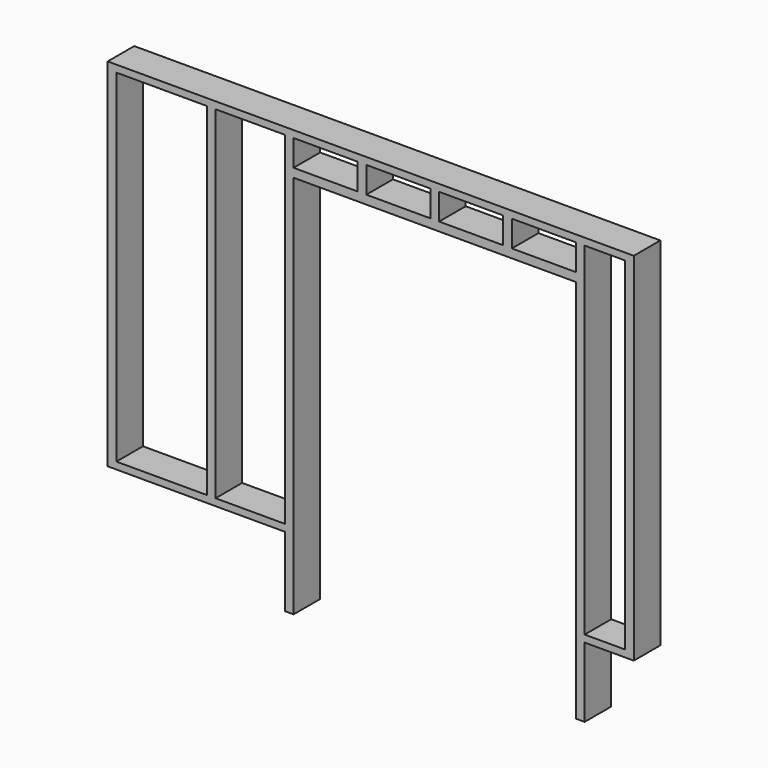
from build123d import *

# Parameters (mm, degrees)
F0_W     = 1014
F0_H     = 40
F1_DEPTH = 190
F0_W_2   = 3011
F2_DEPTH = 190
F3_W     = 50
F3_H     = 1960
F3_H_2   = 150
F0_W_3   = 281
F4_DEPTH = 190


# Not quite as in the source:
# - a feature names something its author has since deleted; it is built from what else it names


with BuildPart() as f1:
    # F0 (on Front) → F1 (new body)
    with BuildSketch(Plane.XZ):
        with Locations((-998.5, 20)):
            Rectangle(F0_W, F0_H)
    extrude(amount=F1_DEPTH)



with BuildPart() as f2:
    # F0 (on Front) → F2 (new body)
    with BuildSketch(Plane.XZ):
        with Locations((0, 2020)):
            Rectangle(F0_W_2, F0_H)
    extrude(amount=F2_DEPTH)


with BuildPart() as f1_1:
    add(f1.part)

    add(f2.part)  # F4 merges F2
    # F3 (on Front) + F0 (on Front) → F4 (join)
    with BuildSketch(Plane.XZ):
        with Locations((1480.5, 1020)):
            Rectangle(F3_W, F3_H)
        Polygon((1224.5, 2000), (1174.5, 2000), (1174.5, 1850), (1174.5, 1800), (1174.5, -400), (1224.5, -400), align=None)
        with Locations((783, 1925)):
            Rectangle(F3_W, F3_H_2)
        with Locations((366.5, 1925)):
            Rectangle(F3_W, F3_H_2)
        with Locations((-50, 1925)):
            Rectangle(F3_W, F3_H_2)
        Polygon((-441.5, -400), (-441.5, 1800), (-441.5, 1850), (-441.5, 2000), (-491.5, 2000), (-491.5, -400), align=None)
        with Locations((-912.9, 1020)):
            Rectangle(F3_W, F3_H)
        with Locations((-1480.5, 1020)):
            Rectangle(F3_W, F3_H)
        Polygon((1174.5, 1800), (1174.5, 1850), (808, 1850), (758, 1850), (391.5, 1850), (341.5, 1850), (-25, 1850), (-75, 1850), (-441.5, 1850), (-441.5, 1800), align=None)
    with BuildSketch(Plane.XZ):
        with Locations((1365, 20)):
            Rectangle(F0_W_3, F0_H)
    extrude(amount=F4_DEPTH)


solid = f1_1.part
